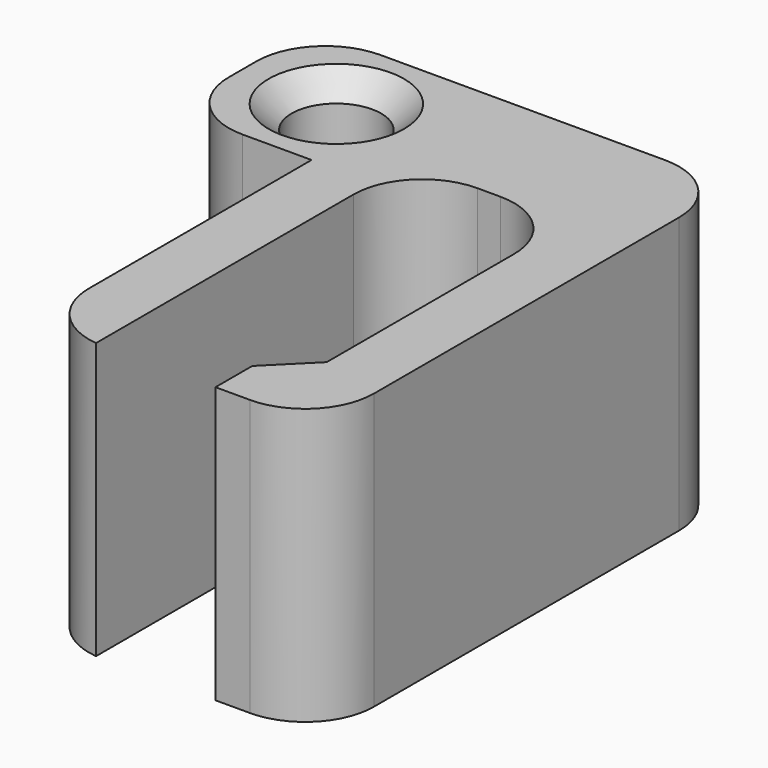
from build123d import *

# Parameters (mm, degrees)
F1_DEPTH     = 6
F2_R         = 0.975
F3_DEPTH     = 6.001
F4_T1_DEPTH  = 6
F4_T3_DEPTH  = 6
F4_T5_DEPTH  = 13.5
F4_T7_DEPTH  = 13.5
F4_T9_DEPTH  = 13.5
F4_T11_DEPTH = 13.5
F4_T13_DEPTH = 13.4624057783
F5_SIZE      = 0.5


# Not quite as in the source:
# - a fillet or chamfer that OpenCascade refuses, or shapes differently, is made with other operations: its cross-section is extruded or revolved along the edge and cut away or added


with BuildPart() as f1:
    # F0 (on Top) → F1 (new body)
    with BuildSketch(Plane.XY):
        Polygon((0, 1.9), (0, 0), (1.35, 0), (1.35, 11.3), (-7.85, 11.3), (-7.85, 7.55), (-4.85, 7.55), (-4.85, 0), (-3.5, 0), (-3.5, 8.5), (0, 8.5), align=None)
        Polygon((-0.9, 0), (0, 0), (0, 1.9), (-0.9, 1), align=None)
    extrude(amount=F1_DEPTH)

    # F2 (on face) → F3 (cut, through all)
    with BuildSketch(Plane.XY.offset(6)):
        with Locations((-5.8098790534, 9.425)):
            Circle(F2_R)
    extrude(amount=-F3_DEPTH, mode=Mode.SUBTRACT)

    # F4: fillet of radius 1.5 on 7 edges, made by hand

    # F4_s2 → F4_t1 (join)
    with BuildSketch(Plane.XY):
        with BuildLine():
            ThreePointArc((0, 7), (-0.4393398282, 8.0606601718), (-1.5, 8.5))
            Line((-1.5, 8.5), (0, 8.5))
            Line((0, 8.5), (0, 7))
        make_face()
    extrude(amount=F4_T1_DEPTH)

    # F4_s4 → F4_t3 (join)
    with BuildSketch(Plane.XY):
        with BuildLine():
            ThreePointArc((-2, 8.5), (-3.0606601718, 8.0606601718), (-3.5, 7))
            Line((-3.5, 7), (-3.5, 8.5))
            Line((-3.5, 8.5), (-2, 8.5))
        make_face()
    extrude(amount=F4_T3_DEPTH)

    # F4_s6 → F4_t5 (cut)
    with BuildSketch(Plane.XY.offset(-3.75)):
        with BuildLine():
            ThreePointArc((1.35, 1.5), (0.9106601718, 0.4393398282), (-0.15, 0))
            Line((-0.15, 0), (1.35, 0))
            Line((1.35, 0), (1.35, 1.5))
        make_face()
    extrude(amount=F4_T5_DEPTH, mode=Mode.SUBTRACT)

    # F4_s8 → F4_t7 (cut)
    with BuildSketch(Plane.XY.offset(-3.75)):
        with BuildLine():
            ThreePointArc((1.35, 9.8), (0.9106601718, 10.8606601718), (-0.15, 11.3))
            Line((-0.15, 11.3), (1.35, 11.3))
            Line((1.35, 11.3), (1.35, 9.8))
        make_face()
    extrude(amount=F4_T7_DEPTH, mode=Mode.SUBTRACT)

    # F4_s10 → F4_t9 (cut)
    with BuildSketch(Plane.XY.offset(-3.75)):
        with BuildLine():
            ThreePointArc((-7.85, 9.8), (-7.4106601718, 10.8606601718), (-6.35, 11.3))
            Line((-6.35, 11.3), (-7.85, 11.3))
            Line((-7.85, 11.3), (-7.85, 9.8))
        make_face()
    extrude(amount=F4_T9_DEPTH, mode=Mode.SUBTRACT)

    # F4_s12 → F4_t11 (cut)
    with BuildSketch(Plane.XY.offset(-3.75)):
        with BuildLine():
            ThreePointArc((-6.35, 7.55), (-7.4106601718, 7.9893398282), (-7.85, 9.05))
            Line((-7.85, 9.05), (-7.85, 7.55))
            Line((-7.85, 7.55), (-6.35, 7.55))
        make_face()
    extrude(amount=F4_T11_DEPTH, mode=Mode.SUBTRACT)

    # F4_s14 → F4_t13 (cut)
    with BuildSketch(Plane.XY.offset(-3.7312028891)):
        with BuildLine():
            ThreePointArc((-3.5, 0), (-4.4624297731, 0.4862505658), (-4.85, 1.4924811557))
            Line((-4.85, 1.4924811557), (-4.85, 0))
            Line((-4.85, 0), (-3.5, 0))
        make_face()
    extrude(amount=F4_T13_DEPTH, mode=Mode.SUBTRACT)

    # F5
    f5_edges = [f1.edges().sort_by_distance(p)[0] for p in [
        (-6.784879, 9.425, 6),
        (-6.784879, 9.425, 0),
    ]]
    chamfer(f5_edges, length=F5_SIZE)


solid = f1.part
